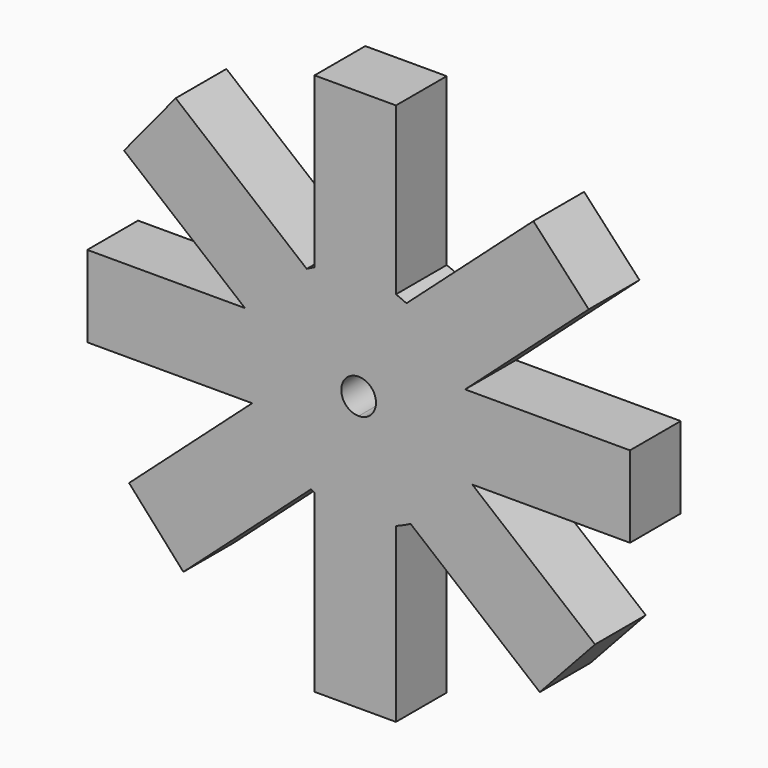
from build123d import *

# Parameters (mm, degrees)
F1_DEPTH = 5.842


with BuildPart() as f1:
    # F0 (on Front) → F1 (new body)
    with BuildSketch(Plane.XZ):
        with BuildLine():
            ThreePointArc((9.5433378796, -2.9874239932), (9.8851752336, -1.5110627392), (10, 0))
            ThreePointArc((10, 0), (9.8508269436, 1.7208162387), (9.4077582946, 3.3902925937))
            Line((9.4077582946, 3.3902925937), (5.7582254442, 0.1224102397))
            Line((5.7582254442, 0.1224102397), (9.5433378796, -2.9874239932))
        make_face()
        with BuildLine():
            ThreePointArc((9.4077582946, 3.3902925937), (9.8508269436, 1.7208162387), (10, 0))
            ThreePointArc((10, 0), (9.8851752336, -1.5110627392), (9.5433378796, -2.9874239932))
            Line((9.5433378796, -2.9874239932), (10.4715017977, -3.75))
            Line((10.4715017977, -3.75), (25, -3.75))
            Line((25, -3.75), (25, 3.75))
            Line((25, 3.75), (9.8094753252, 3.75))
            Line((9.8094753252, 3.75), (9.4077582946, 3.3902925937))
        make_face()
        with BuildLine():
            Line((5.7582254442, 0.1224102397), (9.4077582946, 3.3902925937))
            ThreePointArc((9.4077582946, 3.3902925937), (9.3407348831, 3.57080829), (9.2702481089, 3.75))
            Line((9.2702481089, 3.75), (3.43801843, 3.75))
            Line((3.43801843, 3.75), (3.43801843, 2.0286836526))
            Line((3.43801843, 2.0286836526), (5.7582254442, 0.1224102397))
        make_face()
        with BuildLine():
            ThreePointArc((9.2702481089, 3.75), (9.3407348831, 3.57080829), (9.4077582946, 3.3902925937))
            Line((9.4077582946, 3.3902925937), (9.8094753252, 3.75))
            Line((9.8094753252, 3.75), (9.2702481089, 3.75))
        make_face()
        with BuildLine():
            Line((10.4715017977, -3.75), (9.5433378796, -2.9874239932))
            ThreePointArc((9.5433378796, -2.9874239932), (9.4145172462, -3.3714781657), (9.2702481089, -3.75))
            Line((9.2702481089, -3.75), (10.4715017977, -3.75))
        make_face()
        with BuildLine():
            ThreePointArc((9.2702481089, -3.75), (9.4145172462, -3.3714781657), (9.5433378796, -2.9874239932))
            Line((9.5433378796, -2.9874239932), (5.7582254442, 0.1224102397))
            Line((5.7582254442, 0.1224102397), (3.43801843, -1.9551607454))
            Line((3.43801843, -1.9551607454), (3.43801843, -3.75))
            Line((3.43801843, -3.75), (9.2702481089, -3.75))
        make_face()
        with BuildLine():
            Line((3.43801843, 3.75), (9.2702481089, 3.75))
            ThreePointArc((9.2702481089, 3.75), (7.3200398798, 6.8130034609), (4.4046622613, 8.9776918172))
            Line((4.4046622613, 8.9776918172), (3.43801843, 8.1121349231))
            Line((3.43801843, 8.1121349231), (3.43801843, 3.75))
        make_face()
        with BuildLine():
            ThreePointArc((4.4046622613, 8.9776918172), (7.3200398798, 6.8130034609), (9.2702481089, 3.75))
            Line((9.2702481089, 3.75), (9.8094753252, 3.75))
            Line((9.8094753252, 3.75), (21.1996483638, 13.9490438251))
            Line((21.1996483638, 13.9490438251), (16.0986373051, 19.4487675029))
            Line((16.0986373051, 19.4487675029), (4.4046622613, 8.9776918172))
        make_face()
        Polygon((3.43801843, -1.9551607454), (5.7582254442, 0.1224102397), (3.43801843, 2.0286836526), align=None)
        with BuildLine():
            Line((10.4715017977, -3.75), (9.2702481089, -3.75))
            ThreePointArc((9.2702481089, -3.75), (7.4631867576, -6.6558878763), (4.7822119792, -8.7823942399))
            Line((4.7822119792, -8.7823942399), (16.6882236685, -18.5643289542))
            Line((16.6882236685, -18.5643289542), (21.7797240627, -13.0407931571))
            Line((21.7797240627, -13.0407931571), (10.4715017977, -3.75))
        make_face()
        with BuildLine():
            ThreePointArc((4.7822119792, -8.7823942399), (7.4631867576, -6.6558878763), (9.2702481089, -3.75))
            Line((9.2702481089, -3.75), (3.43801843, -3.75))
            Line((3.43801843, -3.75), (3.43801843, -7.6780098428))
            Line((3.43801843, -7.6780098428), (4.7822119792, -8.7823942399))
        make_face()
        with BuildLine():
            Line((3.43801843, 8.1121349231), (4.4046622613, 8.9776918172))
            ThreePointArc((4.4046622613, 8.9776918172), (3.926766698, 9.1967659152), (3.43801843, 9.3904222096))
            Line((3.43801843, 9.3904222096), (3.43801843, 8.1121349231))
        make_face()
        Polygon((1.3429305817, 3.75), (3.43801843, 3.75), (3.43801843, 8.1121349231), (-0.1050080786, 4.9396209927), align=None)
        Polygon((3.43801843, 2.0286836526), (3.43801843, 3.75), (1.3429305817, 3.75), align=None)
        Polygon((1.4335629107, -3.75), (3.43801843, -1.9551607454), (3.43801843, 2.0286836526), (1.3429305817, 3.75), (-1.4335629107, 3.75), (-4.06198157, 1.3964486531), (-4.06198157, -1.5160378684), (-1.3429305817, -3.75), align=None)
        with BuildLine():
            ThreePointArc((0, 1.6), (1.1313708499, 1.1313708499), (1.6, 0))
            ThreePointArc((1.6, 0), (1.1313708499, -1.1313708499), (0, -1.6))
            ThreePointArc((0, -1.6), (-1.6, 0), (0, 1.6))
        make_face(mode=Mode.SUBTRACT)
        Polygon((3.43801843, -3.75), (3.43801843, -1.9551607454), (1.4335629107, -3.75), align=None)
        with BuildLine():
            ThreePointArc((3.43801843, -9.3904222096), (4.1213434094, -9.1112308994), (4.7822119792, -8.7823942399))
            Line((4.7822119792, -8.7823942399), (3.43801843, -7.6780098428))
            Line((3.43801843, -7.6780098428), (3.43801843, -9.3904222096))
        make_face()
        Polygon((3.43801843, -7.6780098428), (3.43801843, -3.75), (1.4335629107, -3.75), (0.1050080786, -4.9396209927), align=None)
        with BuildLine():
            Line((3.43801843, 8.1121349231), (3.43801843, 9.3904222096))
            ThreePointArc((3.43801843, 9.3904222096), (-0.3365719222, 9.9943343621), (-4.06198157, 9.1378501698))
            Line((-4.06198157, 9.1378501698), (-4.06198157, 8.190655627))
            Line((-4.06198157, 8.190655627), (-0.1050080786, 4.9396209927))
            Line((-0.1050080786, 4.9396209927), (3.43801843, 8.1121349231))
        make_face()
        with BuildLine():
            ThreePointArc((-4.06198157, 9.1378501698), (-0.3365719222, 9.9943343621), (3.43801843, 9.3904222096))
            Line((3.43801843, 9.3904222096), (3.43801843, 24.7108984739))
            Line((3.43801843, 24.7108984739), (-4.06198157, 24.7108984739))
            Line((-4.06198157, 24.7108984739), (-4.06198157, 9.1378501698))
        make_face()
        Polygon((-1.4335629107, 3.75), (1.3429305817, 3.75), (-0.1050080786, 4.9396209927), align=None)
        Polygon((0.1050080786, -4.9396209927), (1.4335629107, -3.75), (-1.3429305817, -3.75), align=None)
        with BuildLine():
            Line((3.43801843, -25.2891015261), (3.43801843, -9.3904222096))
            ThreePointArc((3.43801843, -9.3904222096), (-0.3365719222, -9.9943343621), (-4.06198157, -9.1378501698))
            Line((-4.06198157, -9.1378501698), (-4.06198157, -25.2891015261))
            Line((-4.06198157, -25.2891015261), (3.43801843, -25.2891015261))
        make_face()
        with BuildLine():
            ThreePointArc((-4.06198157, -9.1378501698), (-0.3365719222, -9.9943343621), (3.43801843, -9.3904222096))
            Line((3.43801843, -9.3904222096), (3.43801843, -7.6780098428))
            Line((3.43801843, -7.6780098428), (0.1050080786, -4.9396209927))
            Line((0.1050080786, -4.9396209927), (-4.06198157, -8.6708470153))
            Line((-4.06198157, -8.6708470153), (-4.06198157, -9.1378501698))
        make_face()
        with BuildLine():
            Line((-4.06198157, 8.190655627), (-4.06198157, 9.1378501698))
            ThreePointArc((-4.06198157, 9.1378501698), (-4.4256668552, 8.9673559585), (-4.7822119792, 8.7823942399))
            Line((-4.7822119792, 8.7823942399), (-4.06198157, 8.190655627))
        make_face()
        Polygon((-1.4335629107, 3.75), (-0.1050080786, 4.9396209927), (-4.06198157, 8.190655627), (-4.06198157, 3.75), align=None)
        Polygon((-4.06198157, 1.3964486531), (-1.4335629107, 3.75), (-4.06198157, 3.75), align=None)
        Polygon((-4.06198157, -8.6708470153), (0.1050080786, -4.9396209927), (-1.3429305817, -3.75), (-4.06198157, -3.75), align=None)
        Polygon((-4.06198157, -3.75), (-1.3429305817, -3.75), (-4.06198157, -1.5160378684), align=None)
        with BuildLine():
            ThreePointArc((-4.4046622613, -8.9776918172), (-4.2340792524, -9.0593914191), (-4.06198157, -9.1378501698))
            Line((-4.06198157, -9.1378501698), (-4.06198157, -8.6708470153))
            Line((-4.06198157, -8.6708470153), (-4.4046622613, -8.9776918172))
        make_face()
        with BuildLine():
            Line((-4.06198157, 8.190655627), (-4.7822119792, 8.7823942399))
            ThreePointArc((-4.7822119792, 8.7823942399), (-7.4631867576, 6.6558878763), (-9.2702481089, 3.75))
            Line((-9.2702481089, 3.75), (-4.06198157, 3.75))
            Line((-4.06198157, 3.75), (-4.06198157, 8.190655627))
        make_face()
        with BuildLine():
            ThreePointArc((-9.2702481089, 3.75), (-7.4631867576, 6.6558878763), (-4.7822119792, 8.7823942399))
            Line((-4.7822119792, 8.7823942399), (-16.8534109154, 18.700046179))
            Line((-16.8534109154, 18.700046179), (-21.6145368158, 12.9050759323))
            Line((-21.6145368158, 12.9050759323), (-10.4715017977, 3.75))
            Line((-10.4715017977, 3.75), (-9.2702481089, 3.75))
        make_face()
        with BuildLine():
            Line((-5.7582254442, -0.1224102397), (-4.06198157, 1.3964486531))
            Line((-4.06198157, 1.3964486531), (-4.06198157, 3.75))
            Line((-4.06198157, 3.75), (-9.2702481089, 3.75))
            ThreePointArc((-9.2702481089, 3.75), (-9.4145172462, 3.3714781657), (-9.5433378796, 2.9874239932))
            Line((-9.5433378796, 2.9874239932), (-5.7582254442, -0.1224102397))
        make_face()
        Polygon((-4.06198157, -1.5160378684), (-4.06198157, 1.3964486531), (-5.7582254442, -0.1224102397), align=None)
        with BuildLine():
            Line((-4.4046622613, -8.9776918172), (-4.06198157, -8.6708470153))
            Line((-4.06198157, -8.6708470153), (-4.06198157, -3.75))
            Line((-4.06198157, -3.75), (-9.2702481089, -3.75))
            ThreePointArc((-9.2702481089, -3.75), (-7.3200398798, -6.8130034609), (-4.4046622613, -8.9776918172))
        make_face()
        with BuildLine():
            Line((-9.2702481089, -3.75), (-4.06198157, -3.75))
            Line((-4.06198157, -3.75), (-4.06198157, -1.5160378684))
            Line((-4.06198157, -1.5160378684), (-5.7582254442, -0.1224102397))
            Line((-5.7582254442, -0.1224102397), (-9.4077582946, -3.3902925937))
            ThreePointArc((-9.4077582946, -3.3902925937), (-9.3407348831, -3.57080829), (-9.2702481089, -3.75))
        make_face()
        with BuildLine():
            Line((-16.1475948178, -19.4926052757), (-4.4046622613, -8.9776918172))
            ThreePointArc((-4.4046622613, -8.9776918172), (-7.3200398798, -6.8130034609), (-9.2702481089, -3.75))
            Line((-9.2702481089, -3.75), (-9.8094753252, -3.75))
            Line((-9.8094753252, -3.75), (-21.1506908511, -13.9052060523))
            Line((-21.1506908511, -13.9052060523), (-16.1475948178, -19.4926052757))
        make_face()
        with BuildLine():
            ThreePointArc((-9.5433378796, 2.9874239932), (-9.4145172462, 3.3714781657), (-9.2702481089, 3.75))
            Line((-9.2702481089, 3.75), (-10.4715017977, 3.75))
            Line((-10.4715017977, 3.75), (-9.5433378796, 2.9874239932))
        make_face()
        with BuildLine():
            Line((-9.4077582946, -3.3902925937), (-5.7582254442, -0.1224102397))
            Line((-5.7582254442, -0.1224102397), (-9.5433378796, 2.9874239932))
            ThreePointArc((-9.5433378796, 2.9874239932), (-9.9977411832, -0.2125352519), (-9.4077582946, -3.3902925937))
        make_face()
        with BuildLine():
            Line((-9.8094753252, -3.75), (-9.2702481089, -3.75))
            ThreePointArc((-9.2702481089, -3.75), (-9.3407348831, -3.57080829), (-9.4077582946, -3.3902925937))
            Line((-9.4077582946, -3.3902925937), (-9.8094753252, -3.75))
        make_face()
        with BuildLine():
            ThreePointArc((-9.4077582946, -3.3902925937), (-9.9977411832, -0.2125352519), (-9.5433378796, 2.9874239932))
            Line((-9.5433378796, 2.9874239932), (-10.4715017977, 3.75))
            Line((-10.4715017977, 3.75), (-25, 3.75))
            Line((-25, 3.75), (-25, -3.75))
            Line((-25, -3.75), (-9.8094753252, -3.75))
            Line((-9.8094753252, -3.75), (-9.4077582946, -3.3902925937))
        make_face()
    extrude(amount=F1_DEPTH)


solid = f1.part
